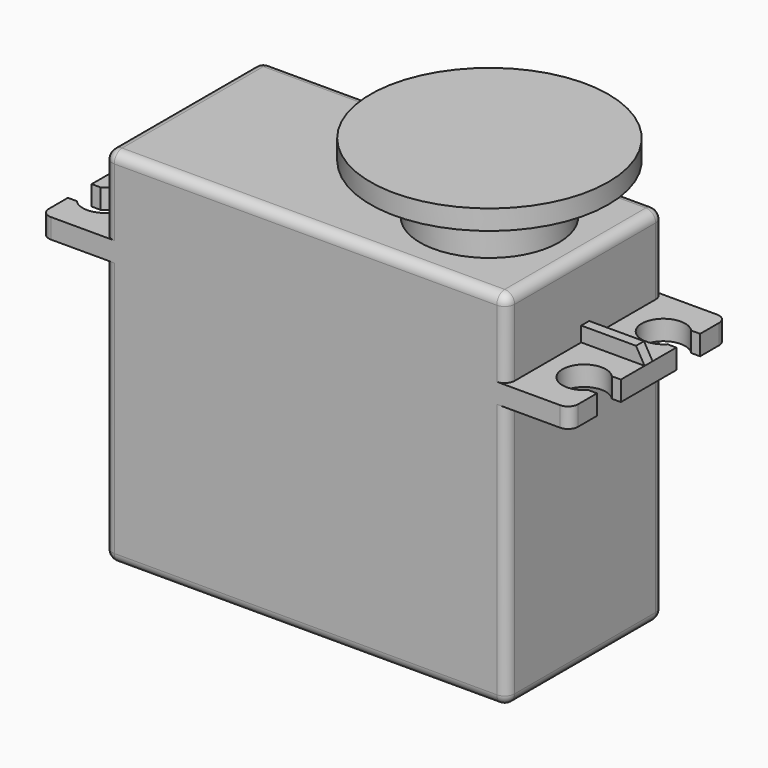
from build123d import *

# Parameters (mm, degrees)
F1_W              = 40.6
F1_H              = 19.8
F2_DEPTH          = 36.6
F3_R              = 7
F4_DEPTH          = 2.5
F5_R              = 4
F6_DEPTH          = 2.5
F7_R              = 12
F8_DEPTH          = 2
F10_W             = 6.4
F10_H             = 19.8
F11_DEPTH         = 2
F13_DEPTH         = 4
F13_COPIES2_COUNT = 2
F14_R             = 1
F16_DEPTH         = 0.5


# Not quite as in the source:
# - a pattern or mirror of a feature is missing from the dataset's text; its kind, count and spacing are read off the source's solid


with BuildPart() as f2:
    # F1 (on Top) → F2 (new body)
    with BuildSketch(Plane.XY):
        Rectangle(F1_W, F1_H)
    extrude(amount=F2_DEPTH)

    # F3 (on face) → F4 (join)
    with BuildSketch(Plane.XY.offset(36.6)):
        with Locations((10.64, 0)):
            Circle(F3_R)
    extrude(amount=F4_DEPTH)

    # F5 (on face) → F6 (join)
    with BuildSketch(Plane.XY.offset(39.1)):
        with Locations((10.64, 0)):
            Circle(F5_R)
    extrude(amount=F6_DEPTH)

    # F7 (on face) → F8 (join)
    with BuildSketch(Plane.XY.offset(41.6)):
        with Locations((10.64, 0)):
            Circle(F7_R)
    extrude(amount=F8_DEPTH)

    # F10 (on offset) → F11 (join)
    with BuildSketch(Plane.XY.offset(26.8)):
        with Locations((23.5, 0)):
            Rectangle(F10_W, F10_H)
    f11 = extrude(amount=F11_DEPTH)

    # F11_copies: F11 across plane
    add(f11.mirror(Plane(origin=(0, 0, 0), x_dir=(0, 0, -1), z_dir=(-1, 0, 0))))

    # F12 (on offset) → F13 (cut)
    with BuildSketch(Plane.XY.offset(26.8)):
        with BuildLine():
            Line((26.7, -3.5), (25.7956503376, -3.5))
            ThreePointArc((25.7956503376, -3.5), (22.01, -5), (25.7956503376, -6.5))
            Line((25.7956503376, -6.5), (26.7, -6.5))
            Line((26.7, -6.5), (26.7, -3.5))
        make_face()
    f13 = extrude(amount=F13_DEPTH, mode=Mode.SUBTRACT)

    # F13_copies: F13 across plane
    add(f13.mirror(Plane(origin=(0, 0, 0), x_dir=(0, 0, -1), z_dir=(-1, 0, 0))), mode=Mode.SUBTRACT)

    # F13_copies1: F13 across plane
    add(f13.mirror(Plane.ZX), mode=Mode.SUBTRACT)

    # F13_copies2: F13 ×2 about axis
    f13_copies2_axis = Axis((0, 0, 0), (0, 0, 1))
    for i in range(1, F13_COPIES2_COUNT):
        add(f13.rotate(f13_copies2_axis, i * 360 / F13_COPIES2_COUNT), mode=Mode.SUBTRACT)

    # F14
    f14_edges = [f2.edges().sort_by_distance(p)[0] for p in [
        (-20.3, -9.9, 13.4),
        (0, -9.9, 0),
        (-20.3, 0, 0),
        (-20.3, 9.9, 13.4),
        (0, 9.9, 0),
        (20.3, 0, 0),
        (20.3, 9.9, 13.4),
        (20.3, -9.9, 13.4),
        (-20.3, 0, 36.6),
        (0, 9.9, 36.6),
        (0, -9.9, 36.6),
        (20.3, -9.9, 32.7),
        (20.3, 0, 36.6),
        (20.3, 9.9, 32.7),
        (26.7, -9.9, 27.8),
        (26.7, 9.9, 27.8),
        (-20.3, 9.9, 32.7),
        (-26.7, 9.9, 27.8),
        (-20.3, -9.9, 32.7),
        (-26.7, -9.9, 27.8),
    ]]
    fillet(f14_edges, radius=F14_R)

    # F15 (on Front) → F16 (join, symmetric)
    with BuildSketch(Plane.XZ):
        Polygon((26.7, 28.8), (25.8339745962, 30.3), (20.3, 30.3), (20.3, 28.8), align=None)
    f16 = extrude(amount=F16_DEPTH, both=True)

    # F16_copies: F16 across plane
    add(f16.mirror(Plane(origin=(0, 0, 0), x_dir=(0, 0, -1), z_dir=(-1, 0, 0))))


solid = f2.part
